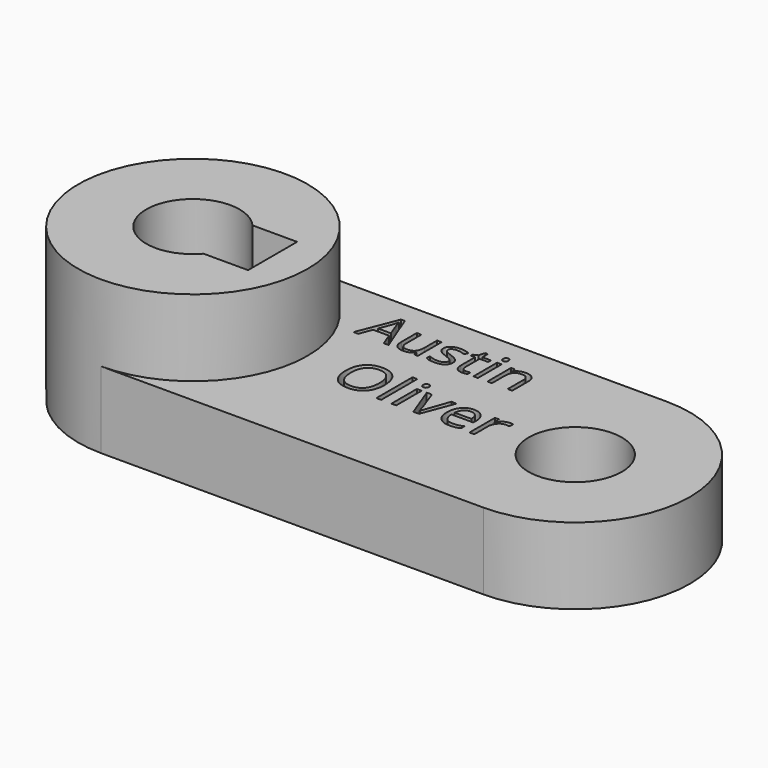
from build123d import *

# Parameters (mm, degrees)
F0_R           = 15.4871514481
F1_DEPTH       = 25.4
F2_DEPTH       = 50.8
F3_TEXT_SIZE   = 18.4112409544
F3_TEXT_SIZE_2 = 19.7263324582
F4_DEPTH       = 12.7


# Not quite as in the source:
# - Text() gives the source's letters only with a copy of the font that has no kerning and outlines rounded to 1/6400 em; it was checked with that copy


with BuildPart() as f1:
    # F0 (on Top) → F1 (new body)
    with BuildSketch(Plane.XY):
        with BuildLine():
            ThreePointArc((0, 38.1), (26.9407683632, 26.9407683632), (38.1, 0))
            ThreePointArc((38.1, 0), (26.9407683632, -26.9407683632), (0, -38.1))
            Line((0, -38.1), (127, -38.1))
            ThreePointArc((127, -38.1), (88.9, 0), (127, 38.1))
            Line((127, 38.1), (0, 38.1))
        make_face()
        with BuildLine():
            ThreePointArc((165.1, 0), (153.9407683632, 26.9407683632), (127, 38.1))
            ThreePointArc((127, 38.1), (88.9, 0), (127, -38.1))
            ThreePointArc((127, -38.1), (153.9407683632, -26.9407683632), (165.1, 0))
        make_face()
        with Locations((127, 0)):
            Circle(F0_R, mode=Mode.SUBTRACT)
    extrude(amount=F1_DEPTH)

    # F0 (on Top) → F2 (join)
    with BuildSketch(Plane.XY):
        with BuildLine():
            ThreePointArc((0, -38.1), (26.9407683632, -26.9407683632), (38.1, 0))
            ThreePointArc((38.1, 0), (26.9407683632, 26.9407683632), (0, 38.1))
            ThreePointArc((0, 38.1), (-38.1, 0), (0, -38.1))
        make_face()
        with BuildLine():
            ThreePointArc((11.6708769036, -10.1804956794), (-15.4871514481, 0), (11.6708769036, 10.1804956794))
            Line((11.6708769036, 10.1804956794), (26.4621078968, 10.1804956794))
            Line((26.4621078968, 10.1804956794), (26.4621078968, -10.1804956794))
            Line((26.4621078968, -10.1804956794), (11.6708769036, -10.1804956794))
        make_face(mode=Mode.SUBTRACT)
    extrude(amount=F2_DEPTH)

    # F3 (on face) → F4 (cut)
    with BuildSketch(Plane.XY.offset(25.4)):
        with Locations((39.0844345093, 17.8326033056)):
            Text('Austin', F3_TEXT_SIZE, font='Open Sans', text_align=(TextAlign.LEFT, TextAlign.BOTTOM))
        with Locations((49.8155578971, -7.4171009474)):
            Text('Oliver', F3_TEXT_SIZE_2, font='Open Sans', text_align=(TextAlign.LEFT, TextAlign.BOTTOM))
    extrude(amount=-F4_DEPTH, mode=Mode.SUBTRACT)


solid = f1.part
